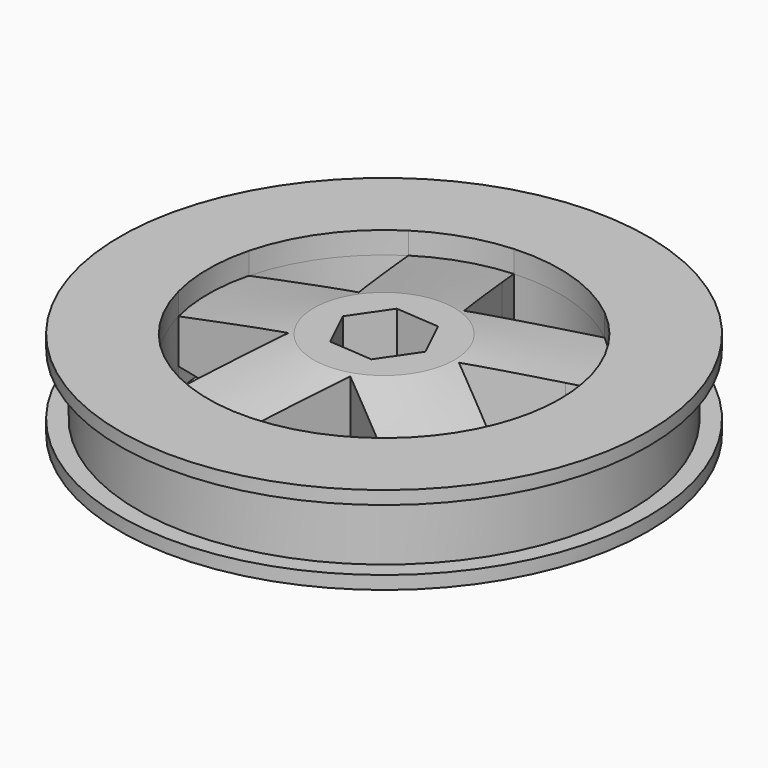
from build123d import *

# Parameters (mm, degrees)
F0_W     = 1.27
F0_H     = 2.2225
F0_W_2   = 7.62
F0_H_2   = 1.5875
F3_DEPTH = 25.4
F6_DEPTH = 6.35


# Not quite as in the source:
# - after a boolean that leaves OpenCascade's solid faulty, fix() repairs it


with BuildPart() as f1:
    # F0 (on Front) → F1 (revolve)
    with BuildSketch(Plane.XZ):
        with Locations((-59.9352485356, 1.11125)):
            Rectangle(F0_W, F0_H)
        with Locations((-59.9352485356, 3.33375)):
            Rectangle(F0_W, F0_H)
        Polygon((-22.4702485356, 5.3975), (-28.8202485356, 5.3975), (-28.8202485356, 3.81), (-28.8202485356, 2.2225), (-22.4702485356, 2.2225), align=None)
        with Locations((-32.6302485356, 3.01625)):
            Rectangle(F0_W_2, F0_H_2)
        Polygon((-36.4402485356, 3.81), (-28.8202485356, 3.81), (-36.4402485356, 5.3975), align=None)
        Polygon((-22.4702485356, -0.9525), (-22.4702485356, 2.2225), (-28.8202485356, 2.2225), (-28.8202485356, 0.635), (-28.8202485356, -0.9525), align=None)
        with Locations((-32.6302485356, 1.42875)):
            Rectangle(F0_W_2, F0_H_2)
        Polygon((-36.4402485356, 2.2225), (-36.4402485356, 3.81), (-36.4402485356, 5.3975), (-38.3452485356, 5.3975), (-38.3452485356, 2.2225), align=None)
        Polygon((-36.4402485356, -0.9525), (-28.8202485356, 0.635), (-36.4402485356, 0.635), align=None)
        Polygon((-36.4402485356, 0.635), (-36.4402485356, 2.2225), (-38.3452485356, 2.2225), (-38.3452485356, -0.9525), (-36.4402485356, -0.9525), align=None)
    revolve(axis=Axis((-41.5202485356, 0, 2.0941267129), (0, 0, 1)))

    add(f1.part.fix(), mode=Mode.REPLACE)

    # F2 (on face) → F3 (cut)
    with BuildSketch(Plane.XY.offset(5.3975)):
        with BuildLine():
            Line((-41.7123280121, 10.8656756712), (-34.9781690591, 8.6776147898))
            Line((-34.9781690591, 8.6776147898), (-33.438209538, 9.7964608733))
            ThreePointArc((-33.438209538, 9.7964608733), (-37.595732707, 12.0784177569), (-42.3005402078, 12.6760066624))
            Line((-42.3005402078, 12.6760066624), (-41.7123280121, 10.8656756712))
        make_face()
        Polygon((-39.8510522546, 5.1372579143), (-34.9781690591, 8.6776147898), (-41.7123280121, 10.8656756712), align=None)
        with BuildLine():
            Line((-51.9134760092, 3.175), (-47.7515368906, 8.9034177569))
            Line((-47.7515368906, 8.9034177569), (-48.3397490863, 10.7137487482))
            ThreePointArc((-48.3397490863, 10.7137487482), (-51.7947643642, 7.4648727041), (-53.8169706598, 3.175))
            Line((-53.8169706598, 3.175), (-51.9134760092, 3.175))
        make_face()
        Polygon((-45.8902611331, 3.175), (-47.7515368906, 8.9034177569), (-51.9134760092, 3.175), align=None)
        with BuildLine():
            Line((-48.3397490863, -10.7137487482), (-47.7515368906, -8.9034177569))
            Line((-47.7515368906, -8.9034177569), (-51.9134760092, -3.175))
            Line((-51.9134760092, -3.175), (-53.8169706598, -3.175))
            ThreePointArc((-53.8169706598, -3.175), (-51.7947643642, -7.4648727041), (-48.3397490863, -10.7137487482))
        make_face()
        Polygon((-51.9134760092, -3.175), (-47.7515368906, -8.9034177569), (-45.8902611331, -3.175), align=None)
        Polygon((-41.7123280121, -10.8656756712), (-34.9781690591, -8.6776147898), (-39.8510522546, -5.1372579143), align=None)
        with BuildLine():
            Line((-33.438209538, -9.7964608733), (-34.9781690591, -8.6776147898))
            Line((-34.9781690591, -8.6776147898), (-41.7123280121, -10.8656756712))
            Line((-41.7123280121, -10.8656756712), (-42.3005402078, -12.6760066624))
            ThreePointArc((-42.3005402078, -12.6760066624), (-37.595732707, -12.0784177569), (-33.438209538, -9.7964608733))
        make_face()
        Polygon((-31.245732707, -3.5403568756), (-31.245732707, 3.5403568756), (-36.1186159026, 0), align=None)
        with BuildLine():
            Line((-29.705773186, 4.659202959), (-31.245732707, 3.5403568756))
            Line((-31.245732707, 3.5403568756), (-31.245732707, -3.5403568756))
            Line((-31.245732707, -3.5403568756), (-29.705773186, -4.659202959))
            ThreePointArc((-29.705773186, -4.659202959), (-29.0435935965, -2.3713037616), (-28.8202485356, 0))
            ThreePointArc((-28.8202485356, 0), (-29.0435935965, 2.3713037616), (-29.705773186, 4.659202959))
        make_face()
    extrude(amount=-F3_DEPTH, mode=Mode.SUBTRACT)

    # F0 (on Front) → F4 (revolve, cut)
    with BuildSketch(Plane.XZ):
        with Locations((-59.9352485356, 3.33375)):
            Rectangle(F0_W, F0_H)
        with Locations((-59.9352485356, 1.11125)):
            Rectangle(F0_W, F0_H)
    revolve(axis=Axis((-41.5202485356, 0, 2.0941267129), (0, 0, 1)), mode=Mode.SUBTRACT)

    add(f1.part.fix(), mode=Mode.REPLACE)

    # F5 (on face) → F6 (join)
    with BuildSketch(Plane.XY.offset(5.3975)):
        with BuildLine():
            Line((-44.6860680874, 0.2412707303), (-42.8942117298, 2.8623155208))
            ThreePointArc((-42.8942117298, 2.8623155208), (-44.1412933261, 1.7918563576), (-44.6860680874, 0.2412707303))
        make_face()
        with BuildLine():
            Line((-43.3121048932, -2.6210447905), (-44.6860680874, 0.2412707303))
            ThreePointArc((-44.6860680874, 0.2412707303), (-44.3825640564, -1.3739631943), (-43.3121048932, -2.6210447905))
        make_face()
        with BuildLine():
            ThreePointArc((-43.3121048932, -2.6210447905), (-41.7615192659, -3.1658195518), (-40.1462853413, -2.8623155208))
            Line((-40.1462853413, -2.8623155208), (-43.3121048932, -2.6210447905))
        make_face()
        with BuildLine():
            ThreePointArc((-40.1462853413, -2.8623155208), (-38.8992037451, -1.7918563576), (-38.3544289838, -0.2412707303))
            Line((-38.3544289838, -0.2412707303), (-40.1462853413, -2.8623155208))
        make_face()
        with BuildLine():
            ThreePointArc((-38.3544289838, -0.2412707303), (-38.3475444778, -0.1207226635), (-38.3452485356, 0))
            ThreePointArc((-38.3452485356, 0), (-38.7122448911, 1.4818031355), (-39.728392178, 2.6210447905))
            Line((-39.728392178, 2.6210447905), (-38.3544289838, -0.2412707303))
        make_face()
        with BuildLine():
            Line((-42.8942117298, 2.8623155208), (-39.728392178, 2.6210447905))
            ThreePointArc((-39.728392178, 2.6210447905), (-41.2789778053, 3.1658195518), (-42.8942117298, 2.8623155208))
        make_face()
    extrude(amount=-F6_DEPTH)


solid = f1.part
